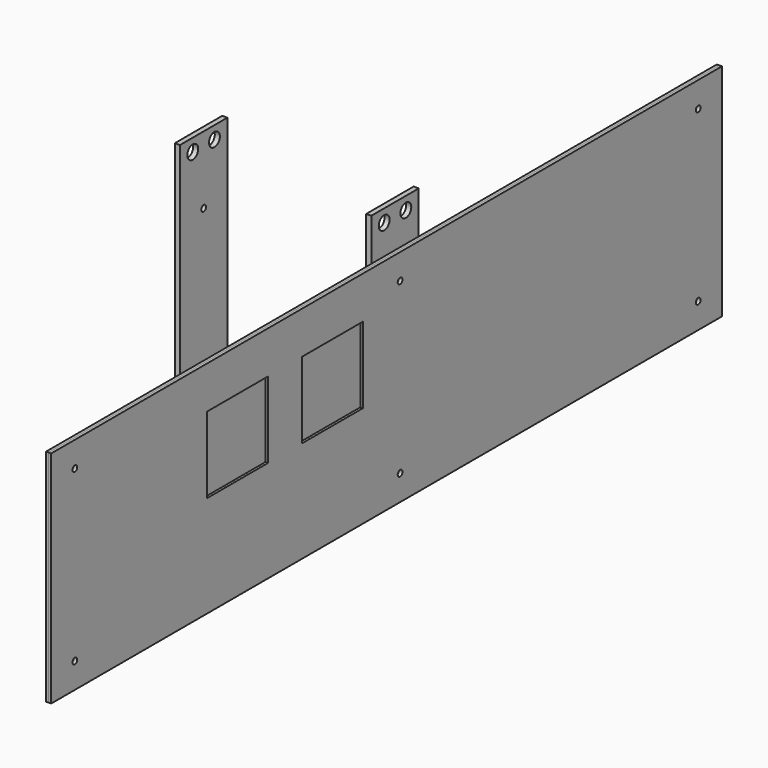
from build123d import *

# Parameters (mm, degrees)
F1_DEPTH  = 35
F2_R      = 3
F3_R      = 5
F4_R      = 4
F5_DEPTH  = 116.001
F6_W      = 495
F6_H      = 130
F7_DEPTH  = 1.5
F8_R      = 1.75
F9_DEPTH  = 117.501
F10_DEPTH = 1.5
F11_W     = 45
F11_H     = 45
F12_DEPTH = 25
F13_W     = 30
F13_H     = 25
F14_DEPTH = 25


with BuildPart() as f1:
    # F0 (on Front) → F1 (new body)
    with BuildSketch(Plane.XZ):
        Polygon((-58, -77.5), (58, -77.5), (58, 77.5), (55, 77.5), (55, -74.5), (-55, -74.5), (-55, 77.5), (-58, 77.5), align=None)
    extrude(amount=F1_DEPTH)

    # F2
    f2_edges = [f1.edges().sort_by_distance(p)[0] for p in [
        (55, -17.5, -74.5),
    ]]
    fillet(f2_edges, radius=F2_R)

    # F3
    f3_edges = [f1.edges().sort_by_distance(p)[0] for p in [
        (-58, -17.5, -77.5),
        (58, -17.5, -77.5),
    ]]
    fillet(f3_edges, radius=F3_R)

    # F4 (on face) → F5 (cut, through all)
    with BuildSketch(Plane(origin=(-58, 0, 0), x_dir=(0, -1, 0), z_dir=(-1, 0, 0))):
        with Locations((9.5, 70)):
            Circle(F4_R)
        with Locations((25.5, 70)):
            Circle(F4_R)
    extrude(amount=-F5_DEPTH, mode=Mode.SUBTRACT)


with BuildPart() as f7:
    # F6 (on face) → F7 (new body)
    with BuildSketch(Plane.YZ.offset(58)):
        with Locations((-27.5, -12.5)):
            Rectangle(F6_W, F6_H)
    extrude(amount=F7_DEPTH)


with BuildPart() as f9_tool:
    # F8 (on face) → F9 (new body, through all)
    with BuildSketch(Plane.YZ.offset(59.5)):
        with Locations((-17.5, 37.5)):
            Circle(F8_R)
        with Locations((-17.5, -62.5)):
            Circle(F8_R)
        with Locations((202.5, -62.5)):
            Circle(F8_R)
        with Locations((202.5, 37.5)):
            Circle(F8_R)
        with Locations((-257.5, 37.5)):
            Circle(F8_R)
        with Locations((-257.5, -62.5)):
            Circle(F8_R)
    extrude(amount=-F9_DEPTH)


with BuildPart() as f1_1:
    add(f1.part)

    # F9: cut by f9_tool
    add(f9_tool.part, mode=Mode.SUBTRACT)


with BuildPart() as f7_1:
    add(f7.part)

    # F9: cut by f9_tool
    add(f9_tool.part, mode=Mode.SUBTRACT)


with BuildPart() as f10:
    # F10 (new): a face of the model
    f10_faces = [f7_1.part.faces().sort_by_distance(p)[0] for p in [
        (59.5, -27.5029929343, -12.5),
    ]]
    extrude(f10_faces, amount=F10_DEPTH)

    # F11 (on face) → F12 (cut)
    with BuildSketch(Plane.YZ.offset(61)):
        with Locations((-67.5, 5)):
            Rectangle(F11_W, F11_H)
        with Locations((-137.5, 5)):
            Rectangle(F11_W, F11_H)
    extrude(amount=-F12_DEPTH, mode=Mode.SUBTRACT)


with BuildPart() as f7_2:
    add(f7_1.part)

    # F13 (on face) → F14 (cut)
    with BuildSketch(Plane(origin=(58, 0, 0), x_dir=(0, -1, 0), z_dir=(-1, 0, 0))):
        with Locations((60, -50)):
            Rectangle(F13_W, F13_H)
    extrude(amount=-F14_DEPTH, mode=Mode.SUBTRACT)


solid = Compound([f1_1.part, f10.part, f7_2.part])
